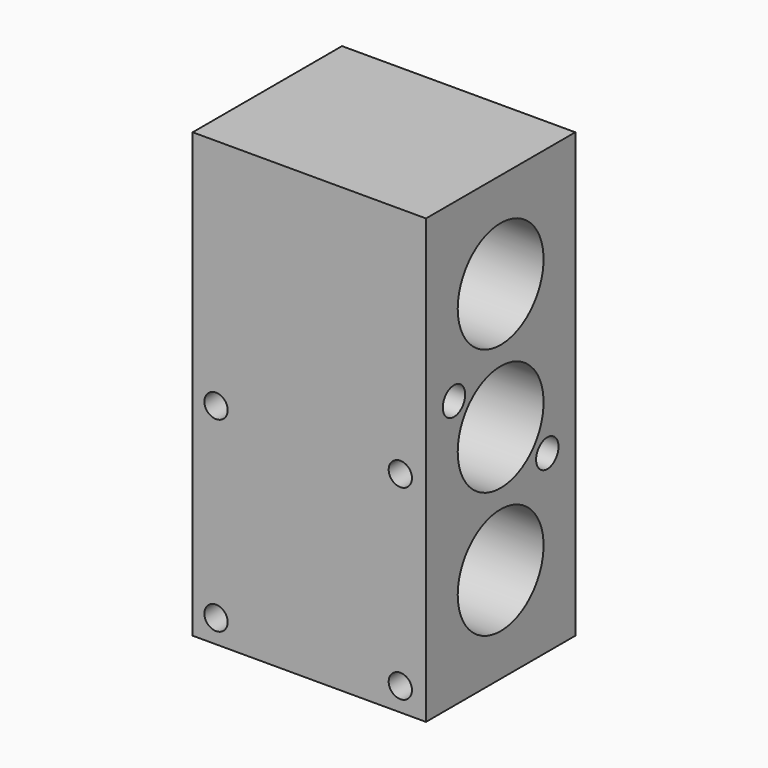
from build123d import *

# Parameters (mm, degrees)
F0_W      = 50
F0_H      = 95
F1_DEPTH  = 40
F2_R      = 2.5
F3_DEPTH  = 18
F4_R      = 11.5
F5_DEPTH  = 20
F7_R      = 11.5
F8_DEPTH  = 50.001
F9_R      = 3
F10_DEPTH = 25


# Not quite as in the source:
# - a pattern or mirror of a feature is missing from the dataset's text; its kind, count and spacing are read off the source's solid


with BuildPart() as f1:
    # F0 (on Front) → F1 (new body)
    with BuildSketch(Plane.XZ):
        with Locations((25, 47.5)):
            Rectangle(F0_W, F0_H)
    extrude(amount=F1_DEPTH)

    # F2 (on face) → F3 (cut)
    with BuildSketch(Plane.XZ.offset(40)):
        with Locations((5, 5)):
            Circle(F2_R)
        with Locations((44.5, 5)):
            Circle(F2_R)
        with Locations((5, 45)):
            Circle(F2_R)
        with Locations((44.5, 45)):
            Circle(F2_R)
    extrude(amount=-F3_DEPTH, mode=Mode.SUBTRACT)

    # F4 (on face) → F5 (cut)
    with BuildSketch(Plane(origin=(0, 0, 0), x_dir=(0, -1, 0), z_dir=(-1, 0, 0))):
        with Locations((20, 74.5)):
            Circle(F4_R)
        with Locations((20, 20.5)):
            Circle(F4_R)
    f5 = extrude(amount=-F5_DEPTH, mode=Mode.SUBTRACT)

    # F5_copies: F5 across plane
    add(f5.mirror(Plane(origin=(25, 0, 0), x_dir=(0, 0, 1), z_dir=(1, 0, 0))), mode=Mode.SUBTRACT)

    # F7 (on face) → F8 (cut, through all)
    with BuildSketch(Plane(origin=(0, 0, 0), x_dir=(0, -1, 0), z_dir=(-1, 0, 0))):
        with Locations((20, 47.5)):
            Circle(F7_R)
    extrude(amount=-F8_DEPTH, mode=Mode.SUBTRACT)

    # F9 (on face) → F10 (cut)
    with BuildSketch(Plane.YZ.offset(50)):
        with Locations((-32.5, 57.5)):
            Circle(F9_R)
        with Locations((-7.5, 37.5)):
            Circle(F9_R)
    extrude(amount=-F10_DEPTH, mode=Mode.SUBTRACT)


solid = f1.part
